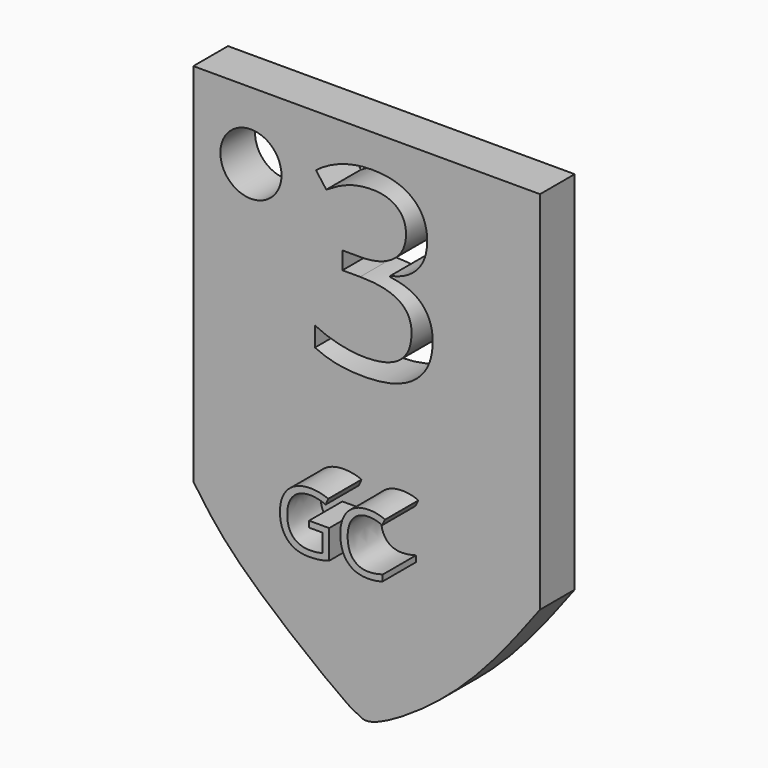
from build123d import *

# Parameters (mm, degrees)
F1_DEPTH     = 2.5
F2_TEXT_SIZE = 14.5323438725
F3_DEPTH     = 2.5
F4_TEXT_SIZE = 4.7803762653
F5_DEPTH     = 4.9
F6_R         = 1.7630968755
F7_DEPTH     = 2.5


# Not quite as in the source:
# - Text() gives the source's letters only with a copy of the font that has no kerning and outlines rounded to 1/6400 em; it was checked with that copy


with BuildPart() as f1:
    # F0 (on Front) → F1 (new body)
    with BuildSketch(Plane.XZ):
        with BuildLine():
            Line((-9.0677969065, 21.1016949298), (-29.0677969065, 21.1016949298))
            Line((-29.0677969065, 21.1016949298), (-29.0677969065, 0))
            add(Edge.make_bspline(
                [(-29.0677969065, 0), (-28.3140110992, -1.0855459531), (-26.5923734921, -3.564919694), (-20.0302019228, -8.6217927094), (-19.58718418, -8.6901896817), (-18.8838166776, -9.2853170347), (-13.5196280215, -5.9395204085), (-10.6388378785, -2.0960431055), (-9.0677969065, 0)],
                knots=[0, 0, 0, 0, 0.1894119624, 0.4326146162, 0.4861029661, 0.5497117355, 0.7544349718, 1, 1, 1, 1], degree=3))
            Line((-9.0677969065, 0), (-9.0677969065, 21.1016949298))
        make_face()
    extrude(amount=F1_DEPTH)

    # F2 (on Front) → F3 (cut, through all)
    with BuildSketch(Plane.XZ):
        with Locations((-22.7163499221, 8.6735151708)):
            Text('3', F2_TEXT_SIZE, font='Open Sans', text_align=(TextAlign.LEFT, TextAlign.BOTTOM))
    extrude(amount=F3_DEPTH, mode=Mode.SUBTRACT)

    # F4 (on Front) → F5 (join)
    with BuildSketch(Plane.XZ):
        with Locations((-22.4409978837, 0)):
            Text('GC', F4_TEXT_SIZE, font='Open Sans', text_align=(TextAlign.LEFT, TextAlign.BOTTOM))
    extrude(amount=F5_DEPTH)

    # F6 (on Front) → F7 (cut, through all)
    with BuildSketch(Plane.XZ):
        with Locations((-25.7451925427, 17.2093547881)):
            Circle(F6_R)
    extrude(amount=F7_DEPTH, mode=Mode.SUBTRACT)


solid = f1.part
